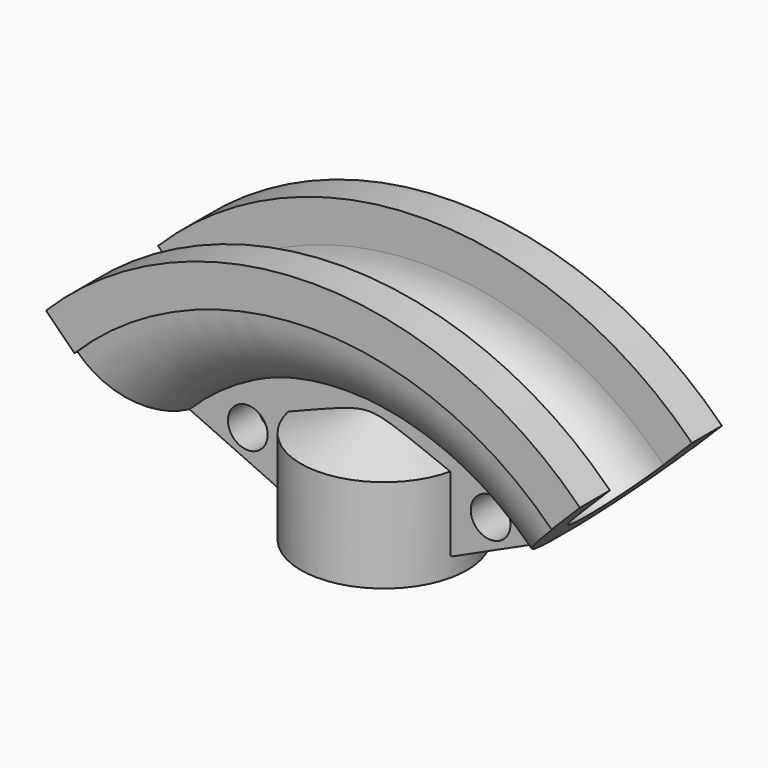
from build123d import *

# Parameters (mm, degrees)
F1_DEPTH      = 10.541
F3_ANGLE_BACK = 45
F3_ANGLE      = 90
F6_R          = 11.303
F7_DEPTH      = 25.4
F8_R          = 25.8445
F9_DEPTH      = 38.1


# Not quite as in the source:
# - a feature names something its author has since deleted; it is built from what else it names


with BuildPart() as f1:
    # F0 (on Front) → F1 (new body, symmetric)
    with BuildSketch(Plane.XZ):
        with BuildLine():
            Line((-102.379978747, 36.2450359051), (-47.371, 11.176))
            Line((-47.371, 11.176), (47.371, 11.176))
            Line((47.371, 11.176), (102.379978747, 36.2450359051))
            ThreePointArc((102.379978747, 36.2450359051), (0, 78.6502618576), (-102.379978747, 36.2450359051))
        make_face()
    extrude(amount=F1_DEPTH, both=True)

    # F4 (on Right) → F5 (revolve)
    with BuildSketch(Plane.YZ):
        Polygon((-47.371, 0), (0, 0), (0, 72.898), (-47.371, 53.34), align=None)
    revolve(axis=Axis((0, 0, 36.449), (0, 0, -1)))

    # F6 (on face) → F7 (cut)
    with BuildSketch(Plane.XZ.offset(10.541)):
        with Locations((-69.1564316947, 37.8521587433)):
            Circle(F6_R)
        with Locations((69.1564316947, 37.8521587433)):
            Circle(F6_R)
    extrude(amount=-F7_DEPTH, mode=Mode.SUBTRACT)

    # F8 (on face) → F9 (cut)
    with BuildSketch(Plane(origin=(0, 0, 0), x_dir=(1, 0, 0), z_dir=(0, 0, -1))):
        Circle(F8_R)
    extrude(amount=-F9_DEPTH, mode=Mode.SUBTRACT)


with BuildPart() as f3:
    # F2 (on Right) → F3 (revolve)
    with BuildSketch(Plane.YZ, mode=Mode.PRIVATE) as f3_sk:
        with BuildLine():
            ThreePointArc((-48.514, 126.0187946151), (-37.8483438872, 95.6689830671), (-10.541, 78.6638))
            Line((-10.541, 78.6638), (10.541, 78.6638))
            ThreePointArc((10.541, 78.6638), (37.8483438872, 95.6689830671), (48.514, 126.0187946151))
            Line((48.514, 126.0187946151), (50.546, 126.0187946151))
            Line((50.546, 126.0187946151), (50.546, 148.8787946151))
            Line((50.546, 148.8787946151), (29.21, 148.8787946151))
            Line((29.21, 148.8787946151), (29.21, 126.0187946151))
            ThreePointArc((29.21, 126.0187946151), (0, 96.8087946151), (-29.21, 126.0187946151))
            Line((-29.21, 126.0187946151), (-29.21, 148.8787946151))
            Line((-29.21, 148.8787946151), (-50.546, 148.8787946151))
            Line((-50.546, 148.8787946151), (-50.546, 126.0187946151))
            Line((-50.546, 126.0187946151), (-48.514, 126.0187946151))
        make_face()
    revolve(f3_sk.sketch.rotate(Axis((0, 7.0290416479, -66.1416), (0, 1, 0)), -F3_ANGLE_BACK), axis=Axis((0, 7.0290416479, -66.1416), (0, 1, 0)), revolution_arc=F3_ANGLE)


solid = Compound([f1.part, f3.part])
